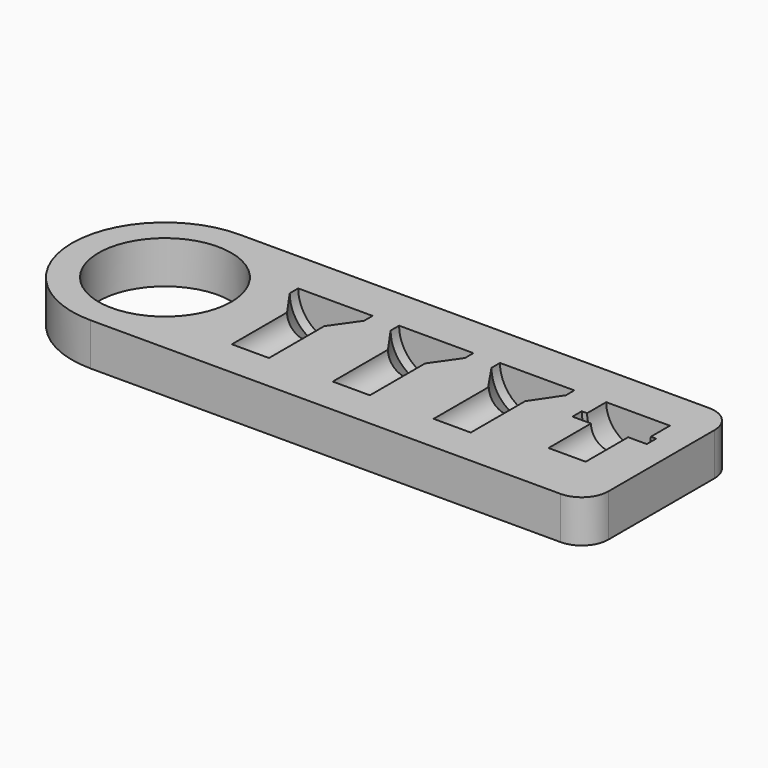
from build123d import *

# Parameters (mm, degrees)
F0_R         = 12.5
F1_DEPTH     = 8
F7_TEXT_SIZE = 5.5555555556
F8_DEPTH     = 1


# Not quite as in the source:
# - Text() gives the source's letters only with a copy of the font that has no kerning and outlines rounded to 1/6400 em; it was checked with that copy


with BuildPart() as f1:
    # F0 (on Top) → F1 (new body)
    with BuildSketch(Plane.XY):
        with BuildLine():
            ThreePointArc((0, 17.5), (5.1256313292, 5.1256313292), (17.5, 0))
            Line((17.5, 0), (106, 0))
            ThreePointArc((106, 0), (109.5355339059, 1.4644660941), (111, 5))
            Line((111, 5), (111, 30))
            ThreePointArc((111, 30), (109.5355339059, 33.5355339059), (106, 35))
            Line((106, 35), (17.5, 35))
            ThreePointArc((17.5, 35), (5.1256313292, 29.8743686708), (0, 17.5))
        make_face()
        with Locations((17.5, 17.5)):
            Circle(F0_R, mode=Mode.SUBTRACT)
    extrude(amount=F1_DEPTH)

    # F2 (on face) → F3 (revolve, cut)
    with BuildSketch(Plane.XY.offset(8)):
        Polygon((105, 27), (99, 27), (99, 22.5), (99, 20.3), (99, 10.3), (102.5, 10.3), (102.5, 20.3), (106, 20.3), (106, 22.5), (105, 22.5), align=None)
    revolve(axis=Axis((99, 15.3, 8), (0, -1, 0)), mode=Mode.SUBTRACT)

    # F2 (on face) → F4 (revolve, cut)
    with BuildSketch(Plane.XY.offset(8)):
        Polygon((87, 27), (80, 27), (80, 25), (80, 20), (80, 7), (83.5, 7), (83.5, 20), (83.6319699883, 20), (87, 25), align=None)
    revolve(axis=Axis((80, 13.5, 8), (0, -1, 0)), mode=Mode.SUBTRACT)

    # F2 (on face) → F5 (revolve, cut)
    with BuildSketch(Plane.XY.offset(8)):
        Polygon((68, 27), (61, 27), (61, 25), (61, 20), (61, 7), (64.5, 7), (64.5, 20), (68, 25), align=None)
    revolve(axis=Axis((61, 13.5, 8), (0, -1, 0)), mode=Mode.SUBTRACT)

    # F2 (on face) → F6 (revolve, cut)
    with BuildSketch(Plane.XY.offset(8)):
        Polygon((49, 27), (42, 27), (42, 25), (42, 20), (42, 7), (45.5, 7), (45.5, 20), (49, 25), align=None)
    revolve(axis=Axis((42, 13.5, 8), (0, -1, 0)), mode=Mode.SUBTRACT)

    # F7 (on face) → F8 (cut)
    with BuildSketch(Plane(origin=(0, 0, 0), x_dir=(1, 0, 0), z_dir=(0, 0, -1))):
        with Locations((30, -9)):
            Text('804, 902', F7_TEXT_SIZE, font='Open Sans', text_align=(TextAlign.LEFT, TextAlign.BOTTOM))
    extrude(amount=-F8_DEPTH, mode=Mode.SUBTRACT)


solid = f1.part
